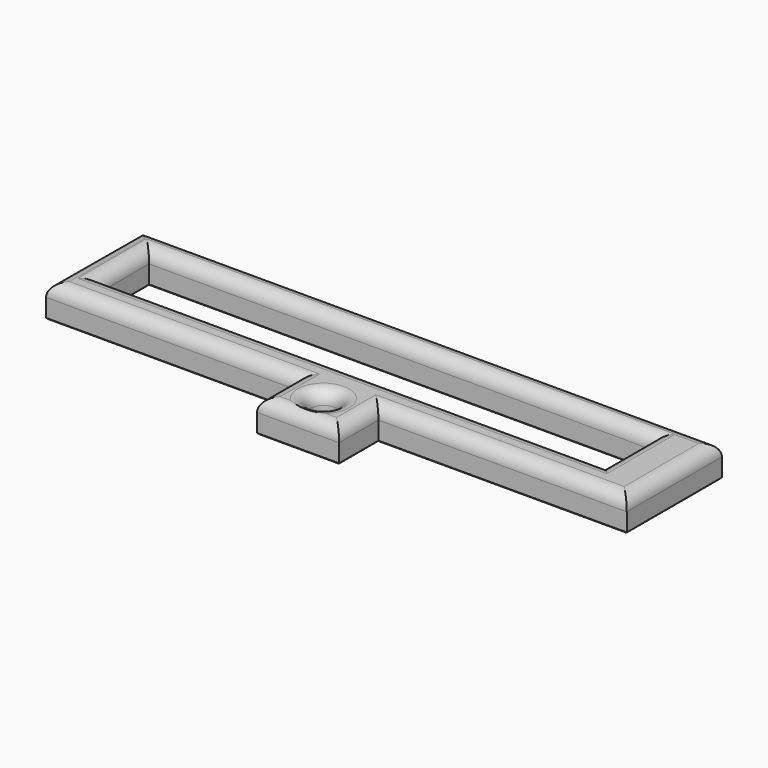
from build123d import *

# Parameters (mm, degrees)
F1_R         = 5.08
F2_DEPTH     = 12.7
F0_W         = 198.4130797122
F0_H         = 23.7392307692
F4_T1_DEPTH  = 254
F4_T3_DEPTH  = 72.2932235662
F4_T5_DEPTH  = 111.3350497574
F4_T7_DEPTH  = 32.0552179203
F4_T9_DEPTH  = 57.7703390416
F4_T11_DEPTH = 110.5876909131
F4_T13_DEPTH = 72.2923076923
F4_T15_DEPTH = 23.7392307692
F4_T17_DEPTH = 198.4130797122
F4_T25_DEPTH = 124.0350497574
F4_T29_DEPTH = 44.7552179203
F4_T36_DEPTH = 44.7552179203
F4_T40_DEPTH = 123.2876909131
F4_T47_DEPTH = 36.4392307692
F4_T51_DEPTH = 211.1130797122
F4_T58_DEPTH = 36.4392307692
F4_T62_DEPTH = 211.1130797122
F4_T69_DEPTH = 211.1130797122
F4_T73_DEPTH = 36.4392307692
F4_T80_DEPTH = 36.4392307692
F4_T84_DEPTH = 211.1130797122
F5_SIZE      = 0.508


# Not quite as in the source:
# - a fillet or chamfer that OpenCascade refuses, or shapes differently, is made with other operations: its cross-section is extruded or revolved along the edge and cut away or added


with BuildPart() as f2:
    # F1 (on face) → F2 (new body)
    with BuildSketch(Plane.XY):
        Polygon((16.1851695208, -22.2859871511), (16.1851695208, -2.9307692308), (-16.1851695208, -2.9307692308), (-16.1851695208, -22.2859871511), (0, -22.2859871511), align=None)
        with Locations((0, -9.8040097783)):
            Circle(F1_R, mode=Mode.SUBTRACT)
    extrude(amount=F2_DEPTH)


with BuildPart() as f2b:
    # F0 (on Top) → F2, piece 2 (new body)
    with BuildSketch(Plane.XY):
        Polygon((114.0728604339, 43.9615384615), (-114.5271395661, 43.9615384615), (-114.8202192782, -2.9307692308), (-16.1851695208, -2.9307692308), (16.1851695208, -2.9307692308), (114.0728604339, -2.9307692308), align=None)
        with Locations((-4.7698304792, 22.4203846154)):
            Rectangle(F0_W, F0_H, mode=Mode.SUBTRACT)
    extrude(amount=F2_DEPTH)


with BuildPart() as f2_1:
    add(f2.part)

    # F3: union F2b
    add(f2b.part)

    # F4: fillet of radius 5.08 on 13 edges, made by hand

    # F4_s2 → F4_t1 (cut)
    with BuildSketch(Plane.YZ.offset(-127.2271395661)):
        with BuildLine():
            ThreePointArc((43.9615384615, 7.62), (42.47364091, 11.2121024484), (38.8815384615, 12.7))
            Line((38.8815384615, 12.7), (43.9615384615, 12.7))
            Line((43.9615384615, 12.7), (43.9615384615, 7.62))
        make_face()
    extrude(amount=F4_T1_DEPTH, mode=Mode.SUBTRACT)

    # F4_s4 → F4_t3 (cut)
    with BuildSketch(Plane(origin=(0.3496520758, 55.9437997302, 0), x_dir=(0, 0, 1), z_dir=(-0.0062499374, -0.999980469, 0))):
        with BuildLine():
            ThreePointArc((7.62, 114.7996595946), (11.2121024484, 113.311762043), (12.7, 109.7196595946))
            Line((12.7, 109.7196595946), (12.7, 114.7996595946))
            Line((12.7, 114.7996595946), (7.62, 114.7996595946))
        make_face()
    extrude(amount=F4_T3_DEPTH, mode=Mode.SUBTRACT)

    # F4_s6 → F4_t5 (cut)
    with BuildSketch(Plane.YZ.offset(-127.5202192782)):
        with BuildLine():
            ThreePointArc((2.1492307692, 12.7), (-1.4428716792, 11.2121024484), (-2.9307692308, 7.62))
            Line((-2.9307692308, 7.62), (-2.9307692308, 12.7))
            Line((-2.9307692308, 12.7), (2.1492307692, 12.7))
        make_face()
    extrude(amount=F4_T5_DEPTH, mode=Mode.SUBTRACT)

    # F4_s8 → F4_t7 (cut)
    with BuildSketch(Plane.XZ.offset(2.9307692308)):
        with BuildLine():
            ThreePointArc((-11.1051695208, 12.7), (-14.6972719692, 11.2121024484), (-16.1851695208, 7.62))
            Line((-16.1851695208, 7.62), (-16.1851695208, 12.7))
            Line((-16.1851695208, 12.7), (-11.1051695208, 12.7))
        make_face()
        with BuildLine():
            ThreePointArc((11.1051695208, 12.7), (14.6972719692, 11.2121024484), (16.1851695208, 7.62))
            Line((16.1851695208, 7.62), (16.1851695208, 12.7))
            Line((16.1851695208, 12.7), (11.1051695208, 12.7))
        make_face()
    extrude(amount=F4_T7_DEPTH, mode=Mode.SUBTRACT)

    # F4_s10 → F4_t9 (cut)
    with BuildSketch(Plane.YZ.offset(-28.8851695208)):
        with BuildLine():
            ThreePointArc((-17.2059871511, 12.7), (-20.7980895995, 11.2121024484), (-22.2859871511, 7.62))
            Line((-22.2859871511, 7.62), (-22.2859871511, 12.7))
            Line((-22.2859871511, 12.7), (-17.2059871511, 12.7))
        make_face()
    extrude(amount=F4_T9_DEPTH, mode=Mode.SUBTRACT)

    # F4_s12 → F4_t11 (cut)
    with BuildSketch(Plane.YZ.offset(16.1851695208)):
        with BuildLine():
            ThreePointArc((2.1492307692, 12.7), (-1.4428716792, 11.2121024484), (-2.9307692308, 7.62))
            Line((-2.9307692308, 7.62), (-2.9307692308, 12.7))
            Line((-2.9307692308, 12.7), (2.1492307692, 12.7))
        make_face()
    extrude(amount=F4_T11_DEPTH, mode=Mode.SUBTRACT)

    # F4_s14 → F4_t13 (cut)
    with BuildSketch(Plane.XZ.offset(-56.6615384615)):
        with BuildLine():
            ThreePointArc((114.0728604339, 7.62), (112.5849628824, 11.2121024484), (108.9928604339, 12.7))
            Line((108.9928604339, 12.7), (114.0728604339, 12.7))
            Line((114.0728604339, 12.7), (114.0728604339, 7.62))
        make_face()
    extrude(amount=F4_T13_DEPTH, mode=Mode.SUBTRACT)

    # F4_s16 → F4_t15 (cut)
    with BuildSketch(Plane.XZ.offset(-34.29)):
        with BuildLine():
            ThreePointArc((-109.0563703353, 12.7), (-105.4642678869, 11.2121024484), (-103.9763703353, 7.62))
            Line((-103.9763703353, 7.62), (-103.9763703353, 12.7))
            Line((-103.9763703353, 12.7), (-109.0563703353, 12.7))
        make_face()
        with BuildLine():
            ThreePointArc((99.5167093769, 12.7), (95.9246069285, 11.2121024484), (94.4367093769, 7.62))
            Line((94.4367093769, 7.62), (94.4367093769, 12.7))
            Line((94.4367093769, 12.7), (99.5167093769, 12.7))
        make_face()
    extrude(amount=F4_T15_DEPTH, mode=Mode.SUBTRACT)

    # F4_s18 → F4_t17 (cut)
    with BuildSketch(Plane.YZ.offset(-103.9763703353)):
        with BuildLine():
            ThreePointArc((39.37, 12.7), (35.7778975516, 11.2121024484), (34.29, 7.62))
            Line((34.29, 7.62), (34.29, 12.7))
            Line((34.29, 12.7), (39.37, 12.7))
        make_face()
        with BuildLine():
            ThreePointArc((5.4707692308, 12.7), (9.0628716792, 11.2121024484), (10.5507692308, 7.62))
            Line((10.5507692308, 7.62), (10.5507692308, 12.7))
            Line((10.5507692308, 12.7), (5.4707692308, 12.7))
        make_face()
    extrude(amount=F4_T17_DEPTH, mode=Mode.SUBTRACT)

    # F4_s19 → F4_t20 (revolve, cut)
    with BuildSketch(Plane.XZ.offset(9.8040097783)):
        with BuildLine():
            ThreePointArc((10.16, 12.7), (6.5678975516, 11.2121024484), (5.08, 7.62))
            Line((5.08, 7.62), (5.08, 12.7))
            Line((5.08, 12.7), (10.16, 12.7))
        make_face()
    revolve(axis=Axis((0, -9.8040097783, 12.7), (0, 0, 1)), mode=Mode.SUBTRACT)


with BuildPart() as f4_tool23:
    # F4_s24 → F4_t25 (new body)
    with BuildSketch(Plane.YZ.offset(-3.4851695208)):
        with BuildLine():
            ThreePointArc((2.1492307692, 12.7), (-1.4428716792, 11.2121024484), (-2.9307692308, 7.62))
            Line((-2.9307692308, 7.62), (-2.9307692308, 12.7))
            Line((-2.9307692308, 12.7), (2.1492307692, 12.7))
        make_face()
    extrude(amount=-F4_T25_DEPTH)

    split(bisect_by=Plane.YZ.offset(-16.1851695208), keep=Keep.TOP)


with BuildPart() as f4_tool27:
    # F4_s28 → F4_t29 (new body)
    with BuildSketch(Plane.XZ.offset(-9.7692307692)):
        with BuildLine():
            ThreePointArc((-11.1051695208, 12.7), (-14.6972719692, 11.2121024484), (-16.1851695208, 7.62))
            Line((-16.1851695208, 7.62), (-16.1851695208, 12.7))
            Line((-16.1851695208, 12.7), (-11.1051695208, 12.7))
        make_face()
    extrude(amount=F4_T29_DEPTH)

    split(bisect_by=Plane.XZ.offset(2.9307692308), keep=Keep.BOTTOM)


with BuildPart() as f4_tool23_1:
    add(f4_tool23.part)

    # F4_t31: intersect F4_tool27
    add(f4_tool27.part, mode=Mode.INTERSECT)


with BuildPart() as f2_2:
    add(f2_1.part)

    # F4_t21: cut F4_tool23
    add(f4_tool23_1.part, mode=Mode.SUBTRACT)


with BuildPart() as f4_tool34:
    # F4_s35 → F4_t36 (new body)
    with BuildSketch(Plane.XZ.offset(34.9859871511)):
        with BuildLine():
            ThreePointArc((11.1051695208, 12.7), (14.6972719692, 11.2121024484), (16.1851695208, 7.62))
            Line((16.1851695208, 7.62), (16.1851695208, 12.7))
            Line((16.1851695208, 12.7), (11.1051695208, 12.7))
        make_face()
    extrude(amount=-F4_T36_DEPTH)

    split(bisect_by=Plane.XZ.offset(2.9307692308), keep=Keep.BOTTOM)


with BuildPart() as f4_tool38:
    # F4_s39 → F4_t40 (new body)
    with BuildSketch(Plane.YZ.offset(126.7728604339)):
        with BuildLine():
            ThreePointArc((2.1492307692, 12.7), (-1.4428716792, 11.2121024484), (-2.9307692308, 7.62))
            Line((-2.9307692308, 7.62), (-2.9307692308, 12.7))
            Line((-2.9307692308, 12.7), (2.1492307692, 12.7))
        make_face()
    extrude(amount=-F4_T40_DEPTH)

    split(bisect_by=Plane.YZ.offset(16.1851695208), keep=Keep.BOTTOM)


with BuildPart() as f4_tool34_1:
    add(f4_tool34.part)

    # F4_t42: intersect F4_tool38
    add(f4_tool38.part, mode=Mode.INTERSECT)


with BuildPart() as f2_3:
    add(f2_2.part)

    # F4_t32: cut F4_tool34
    add(f4_tool34_1.part, mode=Mode.SUBTRACT)


with BuildPart() as f4_tool45:
    # F4_s46 → F4_t47 (new body)
    with BuildSketch(Plane.XZ.offset(2.1492307692)):
        with BuildLine():
            ThreePointArc((-109.0563703353, 12.7), (-105.4642678869, 11.2121024484), (-103.9763703353, 7.62))
            Line((-103.9763703353, 7.62), (-103.9763703353, 12.7))
            Line((-103.9763703353, 12.7), (-109.0563703353, 12.7))
        make_face()
    extrude(amount=-F4_T47_DEPTH)

    split(bisect_by=Plane.XZ.offset(-10.5507692308), keep=Keep.TOP)


with BuildPart() as f4_tool49:
    # F4_s50 → F4_t51 (new body)
    with BuildSketch(Plane.YZ.offset(94.4367093769)):
        with BuildLine():
            ThreePointArc((5.4707692308, 12.7), (9.0628716792, 11.2121024484), (10.5507692308, 7.62))
            Line((10.5507692308, 7.62), (10.5507692308, 12.7))
            Line((10.5507692308, 12.7), (5.4707692308, 12.7))
        make_face()
    extrude(amount=-F4_T51_DEPTH)

    split(bisect_by=Plane.YZ.offset(-103.9763703353), keep=Keep.BOTTOM)


with BuildPart() as f4_tool45_1:
    add(f4_tool45.part)

    # F4_t53: intersect F4_tool49
    add(f4_tool49.part, mode=Mode.INTERSECT)


with BuildPart() as f2_4:
    add(f2_3.part)

    # F4_t43: cut F4_tool45
    add(f4_tool45_1.part, mode=Mode.SUBTRACT)


with BuildPart() as f4_tool56:
    # F4_s57 → F4_t58 (new body)
    with BuildSketch(Plane.XZ.offset(-10.5507692308)):
        with BuildLine():
            ThreePointArc((-109.0563703353, 12.7), (-105.4642678869, 11.2121024484), (-103.9763703353, 7.62))
            Line((-103.9763703353, 7.62), (-103.9763703353, 12.7))
            Line((-103.9763703353, 12.7), (-109.0563703353, 12.7))
        make_face()
    extrude(amount=-F4_T58_DEPTH)

    split(bisect_by=Plane.XZ.offset(-34.29), keep=Keep.BOTTOM)


with BuildPart() as f4_tool60:
    # F4_s61 → F4_t62 (new body)
    with BuildSketch(Plane.YZ.offset(-116.6763703353)):
        with BuildLine():
            ThreePointArc((39.37, 12.7), (35.7778975516, 11.2121024484), (34.29, 7.62))
            Line((34.29, 7.62), (34.29, 12.7))
            Line((34.29, 12.7), (39.37, 12.7))
        make_face()
    extrude(amount=F4_T62_DEPTH)

    split(bisect_by=Plane.YZ.offset(-103.9763703353), keep=Keep.BOTTOM)


with BuildPart() as f4_tool56_1:
    add(f4_tool56.part)

    # F4_t64: intersect F4_tool60
    add(f4_tool60.part, mode=Mode.INTERSECT)


with BuildPart() as f2_5:
    add(f2_4.part)

    # F4_t54: cut F4_tool56
    add(f4_tool56_1.part, mode=Mode.SUBTRACT)


with BuildPart() as f4_tool67:
    # F4_s68 → F4_t69 (new body)
    with BuildSketch(Plane.YZ.offset(-103.9763703353)):
        with BuildLine():
            ThreePointArc((39.37, 12.7), (35.7778975516, 11.2121024484), (34.29, 7.62))
            Line((34.29, 7.62), (34.29, 12.7))
            Line((34.29, 12.7), (39.37, 12.7))
        make_face()
    extrude(amount=F4_T69_DEPTH)

    split(bisect_by=Plane.YZ.offset(94.4367093769), keep=Keep.TOP)


with BuildPart() as f4_tool71:
    # F4_s72 → F4_t73 (new body)
    with BuildSketch(Plane.XZ.offset(-46.99)):
        with BuildLine():
            ThreePointArc((99.5167093769, 12.7), (95.9246069285, 11.2121024484), (94.4367093769, 7.62))
            Line((94.4367093769, 7.62), (94.4367093769, 12.7))
            Line((94.4367093769, 12.7), (99.5167093769, 12.7))
        make_face()
    extrude(amount=F4_T73_DEPTH)

    split(bisect_by=Plane.XZ.offset(-34.29), keep=Keep.BOTTOM)


with BuildPart() as f4_tool67_1:
    add(f4_tool67.part)

    # F4_t75: intersect F4_tool71
    add(f4_tool71.part, mode=Mode.INTERSECT)


with BuildPart() as f2_6:
    add(f2_5.part)

    # F4_t65: cut F4_tool67
    add(f4_tool67_1.part, mode=Mode.SUBTRACT)


with BuildPart() as f4_tool78:
    # F4_s79 → F4_t80 (new body)
    with BuildSketch(Plane.XZ.offset(-34.29)):
        with BuildLine():
            ThreePointArc((99.5167093769, 12.7), (95.9246069285, 11.2121024484), (94.4367093769, 7.62))
            Line((94.4367093769, 7.62), (94.4367093769, 12.7))
            Line((94.4367093769, 12.7), (99.5167093769, 12.7))
        make_face()
    extrude(amount=F4_T80_DEPTH)

    split(bisect_by=Plane.XZ.offset(-10.5507692308), keep=Keep.TOP)


with BuildPart() as f4_tool82:
    # F4_s83 → F4_t84 (new body)
    with BuildSketch(Plane.YZ.offset(107.1367093769)):
        with BuildLine():
            ThreePointArc((5.4707692308, 12.7), (9.0628716792, 11.2121024484), (10.5507692308, 7.62))
            Line((10.5507692308, 7.62), (10.5507692308, 12.7))
            Line((10.5507692308, 12.7), (5.4707692308, 12.7))
        make_face()
    extrude(amount=-F4_T84_DEPTH)

    split(bisect_by=Plane.YZ.offset(94.4367093769), keep=Keep.TOP)


with BuildPart() as f4_tool78_1:
    add(f4_tool78.part)

    # F4_t86: intersect F4_tool82
    add(f4_tool82.part, mode=Mode.INTERSECT)


with BuildPart() as f2_7:
    add(f2_6.part)

    # F4_t76: cut F4_tool78
    add(f4_tool78_1.part, mode=Mode.SUBTRACT)

    # F5
    f5_edges = [f2_7.edges().sort_by_distance(p)[0] for p in [
        (-0.22714, 43.961538, 0),
        (-114.673679, 20.515385, 0),
        (-65.502694, -2.930769, 0),
        (-16.18517, -12.608378, 0),
        (0, -22.285987, 0),
        (16.18517, -12.608378, 0),
        (65.129015, -2.930769, 0),
        (114.07286, 20.515385, 0),
        (-103.97637, 22.420385, 0),
        (-4.76983, 34.29, 0),
        (94.436709, 22.420385, 0),
        (-4.76983, 10.550769, 0),
        (-5.08, -9.80401, 0),
    ]]
    chamfer(f5_edges, length=F5_SIZE)


solid = f2_7.part
